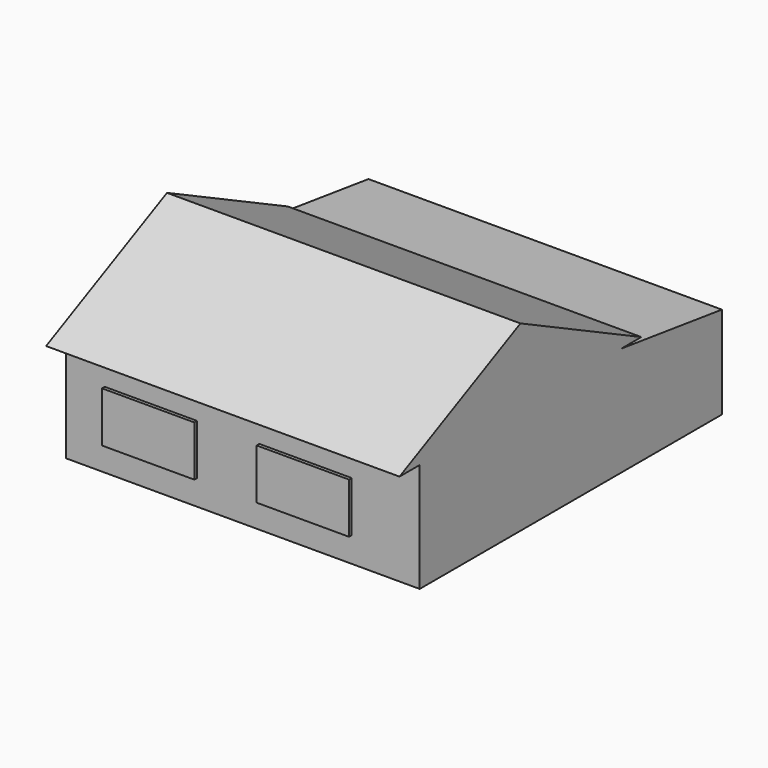
from build123d import *

# Parameters (mm, degrees)
F0_W         = 253.9999981165
F0_H         = 139.6999981165
F0_W_2       = 127.0000127316
F0_H_2       = 109.8118722439
F0_W_3       = 228.6
F0_H_3       = 114.3
F0_W_4       = 381
F0_H_4       = 50.8
F0_W_5       = 101.6
F0_H_5       = 84.4118595123
F0_W_6       = 76.2
F0_H_6       = 177.8
F1_DEPTH     = 1016
F0_TEXT_SIZE = 167.9060773717
F3_DEPTH     = 53.34
F4_DEPTH     = 25.4
F2_W         = 279.4
F2_H         = 152.4
F5_DEPTH     = 10.16
F6_DEPTH     = 10.16
F7_DEPTH     = 12.7


# Not quite as in the source:
# - a feature names something its author has since deleted; it is built from what else it names
# - Text() gives the source's letters only with a copy of the font that has no kerning and outlines rounded to 1/6400 em; it was checked with that copy


with BuildPart() as f1:
    # F0 (on Right) → F1 (new body)
    with BuildSketch(Plane.YZ):
        Polygon((381, 0), (0, 0), (-381, 0), (-381, -279.4), (-304.800003767, -279.4), (-304.800003767, -76.199996233), (-177.799996233, -76.199996233), (-177.799996233, -279.4), (381, -279.4), (381, -50.8), (381, -34.8900556564), align=None)
        with Locations((165.1, -146.05)):
            Rectangle(F0_W, F0_H, mode=Mode.SUBTRACT)
        Polygon((762, -101.6), (381, -50.8), (381, -279.4), (762, -279.4), align=None)
        with Locations((558.8, -178.4579157829)):
            Rectangle(F0_W_2, F0_H_2, mode=Mode.SUBTRACT)
        Polygon((-304.800003767, -279.4), (-381, -279.4), (-381, -330.2), (381, -330.2), (381, -279.4), (-177.799996233, -279.4), (-203.2, -279.4), (-279.4, -279.4), align=None)
        with Locations((165.1, -146.05)):
            Rectangle(F0_W, F0_H)
        with Locations((165.1, -146.05)):
            Rectangle(F0_W_3, F0_H_3, mode=Mode.SUBTRACT)
        Polygon((0, 184.1000467539), (0, 0), (381, 0), align=None)
        Polygon((-381, 0), (0, 0), (0, 184.1000467539), align=None)
        with Locations((165.1, -146.05)):
            Rectangle(F0_W_3, F0_H_3)
        with Locations((571.5, -304.8)):
            Rectangle(F0_W_4, F0_H_4)
        Polygon((762, -50.8), (381, 0), (381, -34.8900556564), (381, -50.8), (762, -101.6), align=None)
        Polygon((-457.2, 0), (-381, 0), (0, 184.1000467539), (0, 222.2000467539), align=None)
        Polygon((0, 184.1000467539), (381, 0), (457.2, 0), (0, 222.2000467539), align=None)
        with Locations((558.8, -178.4579157829)):
            Rectangle(F0_W_2, F0_H_2)
        with Locations((558.8, -178.4579157829)):
            Rectangle(F0_W_5, F0_H_5, mode=Mode.SUBTRACT)
        with Locations((-241.3, -190.5)):
            Rectangle(F0_W_6, F0_H_6)
        Polygon((-304.800003767, -76.199996233), (-304.800003767, -279.4), (-279.4, -279.4), (-279.4, -101.6), (-203.2, -101.6), (-203.2, -279.4), (-177.799996233, -279.4), (-177.799996233, -76.199996233), align=None)
        with Locations((558.8, -178.4579157829)):
            Rectangle(F0_W_5, F0_H_5)
    extrude(amount=F1_DEPTH)

    # F0 (on Right) + F1_face1 (on face) → F3 (join)
    with BuildSketch(Plane.YZ):
        with Locations((328.9575278759, -546.5123653412)):
            Text('Zane', F0_TEXT_SIZE, font='Open Sans', font_style=FontStyle.BOLD, text_align=(TextAlign.LEFT, TextAlign.BOTTOM))
        with BuildLine():
            Line((490.1473621527, -511.5931483128), (490.1473621527, -504.0373748311))
            Line((490.1473621527, -504.0373748311), (480.4665273793, -504.3784340507))
            add(Edge.make_bspline(
                [(480.4665273793, -504.3784340507), (469.5526323501, -504.6932579458), (464.2268614585, -508.3006150768)],
                knots=[0, 0, 0, 1, 1, 1], degree=2))
            add(Edge.make_bspline(
                [(464.2268614585, -508.3006150768), (458.9010905668, -511.9079722079), (458.9010905668, -519.2800984175)],
                knots=[0, 0, 0, 1, 1, 1], degree=2))
            add(Edge.make_bspline(
                [(458.9010905668, -519.2800984175), (458.9010905668, -529.8791695516), (471.0218105271, -529.8791695516)],
                knots=[0, 0, 0, 1, 1, 1], degree=2))
            add(Edge.make_bspline(
                [(471.0218105271, -529.8791695516), (479.7319382908, -529.8791695516), (484.9396502218, -524.868222555)],
                knots=[0, 0, 0, 1, 1, 1], degree=2))
            add(Edge.make_bspline(
                [(484.9396502218, -524.868222555), (490.1473621527, -519.8572755584), (490.1473621527, -511.5931483128)],
                knots=[0, 0, 0, 1, 1, 1], degree=2))
        make_face()
        with BuildLine():
            add(Edge.make_bspline(
                [(701.6565489919, -475.9655775205), (696.986661215, -470.9283951993), (689.0373578644, -470.9283951993)],
                knots=[0, 0, 0, 1, 1, 1], degree=2))
            add(Edge.make_bspline(
                [(689.0373578644, -470.9283951993), (681.0880545139, -470.9283951993), (676.5755786845, -475.9655775205)],
                knots=[0, 0, 0, 1, 1, 1], degree=2))
            add(Edge.make_bspline(
                [(676.5755786845, -475.9655775205), (672.0631028551, -481.0027598416), (671.4072197404, -490.2638294217)],
                knots=[0, 0, 0, 1, 1, 1], degree=2))
            Line((671.4072197404, -490.2638294217), (706.5100840409, -490.2638294217))
            add(Edge.make_bspline(
                [(706.5100840409, -490.2638294217), (706.3264367688, -481.0027598416), (701.6565489919, -475.9655775205)],
                knots=[0, 0, 0, 1, 1, 1], degree=2))
        make_face()
    with BuildSketch(Plane(origin=(1016, 140.0996007109, -116.3858962954), x_dir=(0, 1, 0), z_dir=(1, 0, 0))):
        Polygon((-521.0996007109, -213.8141037046), (621.9003992891, -213.8141037046), (621.9003992891, 65.5858962954), (240.9003992891, 116.3858962954), (317.1003992891, 116.3858962954), (-140.0996007109, 338.5859430493), (-597.2996007109, 116.3858962954), (-521.0996007109, 116.3858962954), align=None)
    extrude(amount=F3_DEPTH)

    # F0 (on Right) → F4 (join)
    with BuildSketch(Plane.YZ):
        with Locations((-241.3, -190.5)):
            Rectangle(F0_W_6, F0_H_6)
    extrude(amount=F4_DEPTH)

    # F2 (on face) → F5 (join)
    with BuildSketch(Plane.XZ.offset(381)):
        with Locations((256.0974226519, -177.8)):
            Rectangle(F2_W, F2_H)
        with Locations((723.9, -177.8)):
            Rectangle(F2_W, F2_H)
    extrude(amount=F5_DEPTH)

    # F0 (on Right) → F6 (join)
    with BuildSketch(Plane.YZ):
        with Locations((165.1, -146.05)):
            Rectangle(F0_W_3, F0_H_3)
        with Locations((558.8, -178.4579157829)):
            Rectangle(F0_W_5, F0_H_5)
    extrude(amount=-F6_DEPTH)

    # F0 (on Right) → F7 (join)
    with BuildSketch(Plane.YZ):
        with Locations((-241.3, -190.5)):
            Rectangle(F0_W_6, F0_H_6)
    extrude(amount=F7_DEPTH)


solid = f1.part
